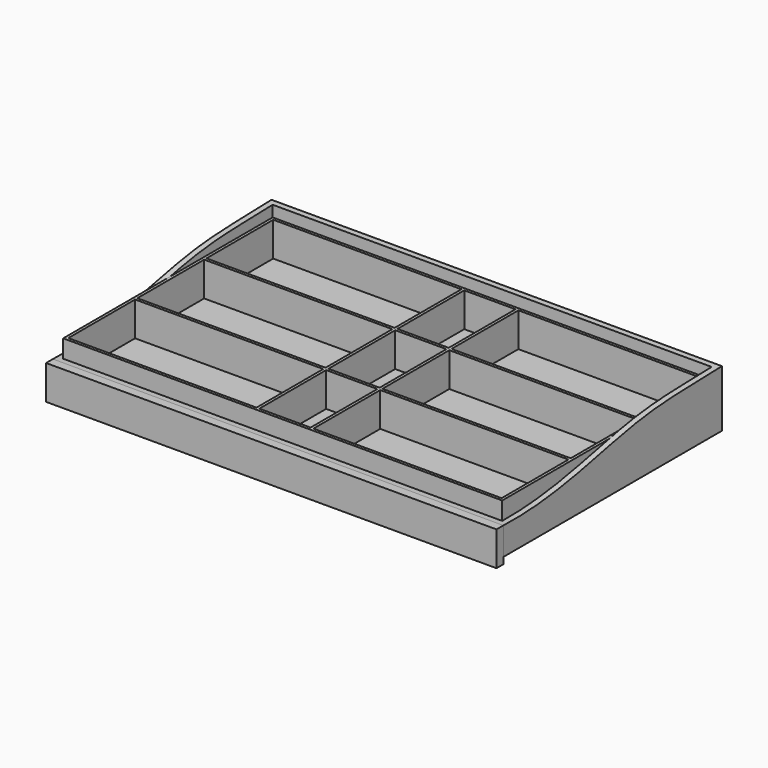
from build123d import *

# Parameters (mm, degrees)
F0_W     = 979.4875
F0_H     = 12.7
F1_DEPTH = 101.6
F2_DEPTH = 25.4
F3_W     = 1004.8875
F3_H     = 609.6
F3_W_2   = 419.89375
F3_H_2   = 186.2666666667
F4_DEPTH = 12.7
F6_DEPTH = 1004.8885
F0_W_2   = 1004.8875
F0_H_2   = 19.05
F7_DEPTH = 36.5125
F8_DEPTH = 39.8145
F0_H_3   = 584.2
F0_W_3   = 419.89375
F0_H_4   = 186.2666666667
F0_W_4   = 114.3
F0_W_5   = 419.8937565804
F9_DEPTH = 76.2


with BuildPart() as f1:
    # F0 (on Top) → F1 (new body)
    with BuildSketch(Plane.XY):
        Polygon((-13.9944232941, 524.1015708923), (-26.6944232941, 524.1015708923), (-26.6944232941, -85.4984291077), (978.1930767059, -85.4984291077), (978.1930767059, 524.1015708923), (965.4930767059, 524.1015708923), (965.4930767059, 511.4015708923), (965.4930767059, -72.7984291077), (-13.9944232941, -72.7984291077), (-13.9944232941, 511.4015708923), align=None)
        with Locations((475.7493267059, 517.7515708923)):
            Rectangle(F0_W, F0_H)
    extrude(amount=F1_DEPTH)

    # F0 (on Top) → F2 (join)
    with BuildSketch(Plane.XY):
        Polygon((-13.9944232941, 524.1015708923), (-26.6944232941, 524.1015708923), (-26.6944232941, -85.4984291077), (978.1930767059, -85.4984291077), (978.1930767059, 524.1015708923), (965.4930767059, 524.1015708923), (965.4930767059, 511.4015708923), (965.4930767059, -72.7984291077), (-13.9944232941, -72.7984291077), (-13.9944232941, 511.4015708923), align=None)
    extrude(amount=-F2_DEPTH)

    # F3 (on face) → F4 (join)
    with BuildSketch(Plane.XY):
        with Locations((475.7493267059, 219.3015708923)):
            Rectangle(F3_W, F3_H)
        with Locations((749.1962017059, 411.918237559)):
            Rectangle(F3_W_2, F3_H_2, mode=Mode.SUBTRACT)
        with Locations((749.1962017059, 411.918237559)):
            Rectangle(F3_W_2, F3_H_2)
    extrude(amount=-F4_DEPTH)

    # F5 (on face) → F6 (cut, through all)
    with BuildSketch(Plane(origin=(-26.6944232941, 0, 0), x_dir=(0, -1, 0), z_dir=(-1, 0, 0))):
        with BuildLine():
            Line((85.4984291077, 101.6), (-524.1015708923, 101.6))
            add(Edge.make_bspline(
                [(-524.1015708923, 101.6), (-454.3829336776, 98.6535593443), (-315.5144360565, 101.3463644472), (-114.7516219339, 48.2200810371), (18.7137848875, 33.9810080981), (85.4984291077, 36.5125)],
                knots=[0, 0, 0, 0, 0.3360631231, 0.6706250277, 1, 1, 1, 1], degree=3))
            Line((85.4984291077, 36.5125), (85.4984291077, 101.6))
        make_face()
    extrude(amount=-F6_DEPTH, mode=Mode.SUBTRACT)


with BuildPart() as f7:
    # F0 (on Top) → F7 (new body)
    with BuildSketch(Plane.XY):
        with Locations((475.7493267059, -95.0234291077)):
            Rectangle(F0_W_2, F0_H_2)
    extrude(amount=F7_DEPTH)

    # F0 (on Top) → F8 (join)
    with BuildSketch(Plane.XY):
        with Locations((475.7493267059, -95.0234291077)):
            Rectangle(F0_W_2, F0_H_2)
    extrude(amount=-F8_DEPTH)


with BuildPart() as f9:
    # F0 (on Top) → F9 (new body)
    with BuildSketch(Plane.XY):
        with Locations((475.7493267059, 219.3015708923)):
            Rectangle(F0_W, F0_H_3)
        with Locations((202.3024517059, 26.6849042257)):
            Rectangle(F0_W_3, F0_H_4, mode=Mode.SUBTRACT)
        with Locations((475.7493267059, 26.6849042257)):
            Rectangle(F0_W_4, F0_H_4, mode=Mode.SUBTRACT)
        with Locations((749.1962017059, 26.6849042257)):
            Rectangle(F0_W_3, F0_H_4, mode=Mode.SUBTRACT)
        with Locations((202.3024517059, 219.3015708923)):
            Rectangle(F0_W_3, F0_H_4, mode=Mode.SUBTRACT)
        with Locations((202.3024517059, 411.918237559)):
            Rectangle(F0_W_3, F0_H_4, mode=Mode.SUBTRACT)
        Polygon((418.5993267059, 312.4349042257), (532.8993267059, 312.4349042257), (532.8993267059, 293.2371660391), (532.8993267059, 126.168237559), (418.5993267059, 126.168237559), align=None, mode=Mode.SUBTRACT)
        with Locations((749.1961984158, 219.3015708923)):
            Rectangle(F0_W_5, F0_H_4, mode=Mode.SUBTRACT)
        with Locations((475.7493267059, 411.918237559)):
            Rectangle(F0_W_4, F0_H_4, mode=Mode.SUBTRACT)
        with Locations((749.1962017059, 411.918237559)):
            Rectangle(F0_W_3, F0_H_4, mode=Mode.SUBTRACT)
    extrude(amount=F9_DEPTH)


solid = Compound([f1.part, f7.part, f9.part])
